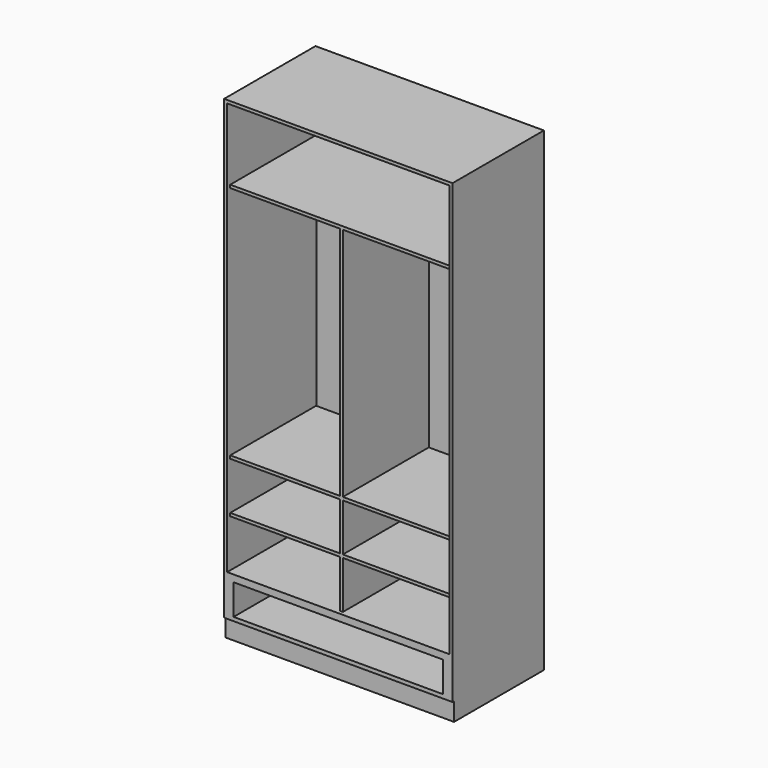
from build123d import *

# Parameters (mm, degrees)
F0_W      = 600
F0_H      = 2496
F1_DEPTH  = 1200
F2_W      = 1200
F2_H      = 96
F3_DEPTH  = 10
F4_W      = 1100
F4_H      = 160
F5_DEPTH  = 580
F7_W      = 1168
F7_H      = 2168
F8_DEPTH  = 586
F9_W      = 1168
F9_H      = 16
F10_DEPTH = 564
F11_W     = 16
F11_H     = 1768
F12_DEPTH = 564
F13_W     = 1168
F13_H     = 16
F14_DEPTH = 564


with BuildPart() as f1:
    # F0 (on Right) → F1 (new body)
    with BuildSketch(Plane.YZ):
        Rectangle(F0_W, F0_H)
    extrude(amount=F1_DEPTH)

    # F2 (on face) → F3 (cut)
    with BuildSketch(Plane.XZ.offset(300)):
        with Locations((600, -1200)):
            Rectangle(F2_W, F2_H)
    extrude(amount=-F3_DEPTH, mode=Mode.SUBTRACT)

    # F4 (on face) → F5 (cut)
    with BuildSketch(Plane.XZ.offset(300)):
        with Locations((600, -1052)):
            Rectangle(F4_W, F4_H)
    extrude(amount=-F5_DEPTH, mode=Mode.SUBTRACT)

    # F7 (on face) → F8 (cut)
    with BuildSketch(Plane.XZ.offset(300)):
        with Locations((600, 148)):
            Rectangle(F7_W, F7_H)
    extrude(amount=-F8_DEPTH, mode=Mode.SUBTRACT)

    # F9 (on offset) → F10 (join)
    with BuildSketch(Plane.XZ.offset(280)):
        with Locations((600, 840)):
            Rectangle(F9_W, F9_H)
    extrude(amount=-F10_DEPTH)

    # F11 (on offset) → F12 (join)
    with BuildSketch(Plane.XZ.offset(280)):
        with Locations((600, -52)):
            Rectangle(F11_W, F11_H)
    extrude(amount=-F12_DEPTH)

    # F13 (on offset) → F14 (join)
    with BuildSketch(Plane.XZ.offset(280)):
        with Locations((600, -678)):
            Rectangle(F13_W, F13_H)
        with Locations((600, -412)):
            Rectangle(F13_W, F13_H)
    extrude(amount=-F14_DEPTH)


solid = f1.part
